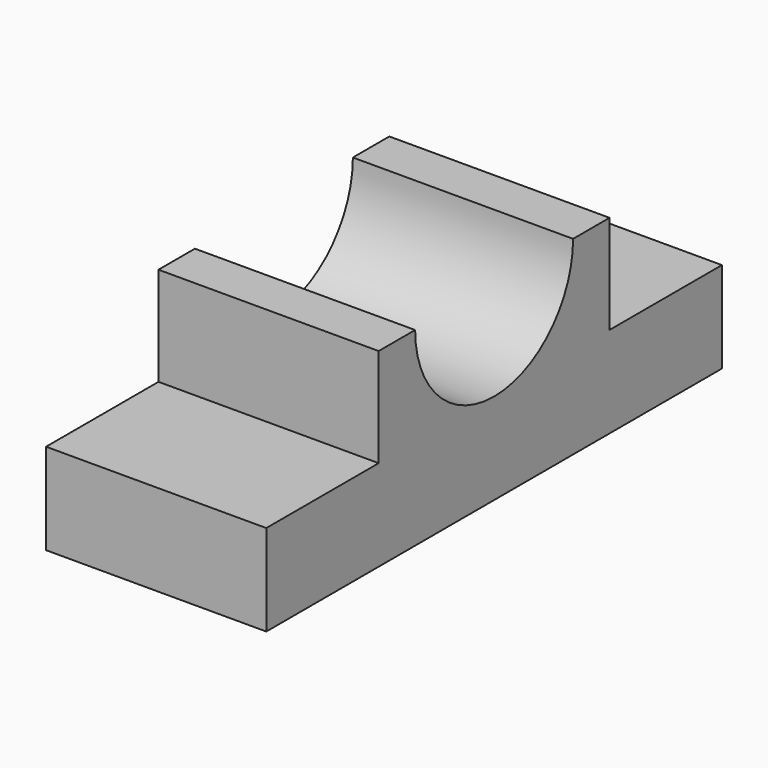
from build123d import *

# Parameters (mm, degrees)
F2_DEPTH = 147.32
F3_DEPTH = 543
F1_R     = 66.04
F4_DEPTH = 147.321


# Not quite as in the source:
# - an extrude ends at something that could not be found from the text; its depth is read off the source's solid


with BuildPart() as f2:
    # F0 (on Right) → F2 (new body)
    with BuildSketch(Plane.YZ):
        Polygon((-227.214354679, -72.635721945), (-227.214354679, -133.595721945), (153.785645321, -133.595721945), (153.785645321, -72.635721945), (59.805645321, -72.635721945), (59.805645321, -6.595721945), (-3.4203693569, -6.595721945), (-97.4624507428, -6.595721945), (-133.234354679, -6.595721945), (-133.234354679, -72.635721945), align=None)
    extrude(amount=F2_DEPTH)

    # F1 (on face) → F3 (cut, through all)
    with BuildSketch(Plane.YZ):
        with BuildLine():
            ThreePointArc((29.3256430177, -6.595721945), (29.3256447452, -6.587001079), (29.325645321, -6.5782802129))
            ThreePointArc((29.325645321, -6.5782802129), (-36.7230755452, 59.4617192113), (-102.7543523758, -6.595721945))
            Line((-102.7543523758, -6.595721945), (-97.4624507428, -6.595721945))
            Line((-97.4624507428, -6.595721945), (-3.4203693569, -6.595721945))
            Line((-3.4203693569, -6.595721945), (29.3256430177, -6.595721945))
        make_face()
    extrude(amount=-F3_DEPTH, mode=Mode.SUBTRACT)

    # F1 (on face) + F2_face (on face) → F4 (cut, through all)
    with BuildSketch(Plane.YZ):
        with Locations((-36.714354679, -6.5782802129)):
            Circle(F1_R)
    with BuildSketch(Plane(origin=(147.32, -36.714354679, -80.6128525046), x_dir=(0, 1, 0), z_dir=(1, 0, 0))):
        Polygon((-190.5, 7.9771305595), (-190.5, -52.9828694405), (190.5, -52.9828694405), (190.5, 7.9771305595), (96.52, 7.9771305595), (96.52, 74.0171305595), (-96.52, 74.0171305595), (-96.52, 7.9771305595), align=None)
    extrude(amount=F4_DEPTH, mode=Mode.SUBTRACT)


solid = f2.part
